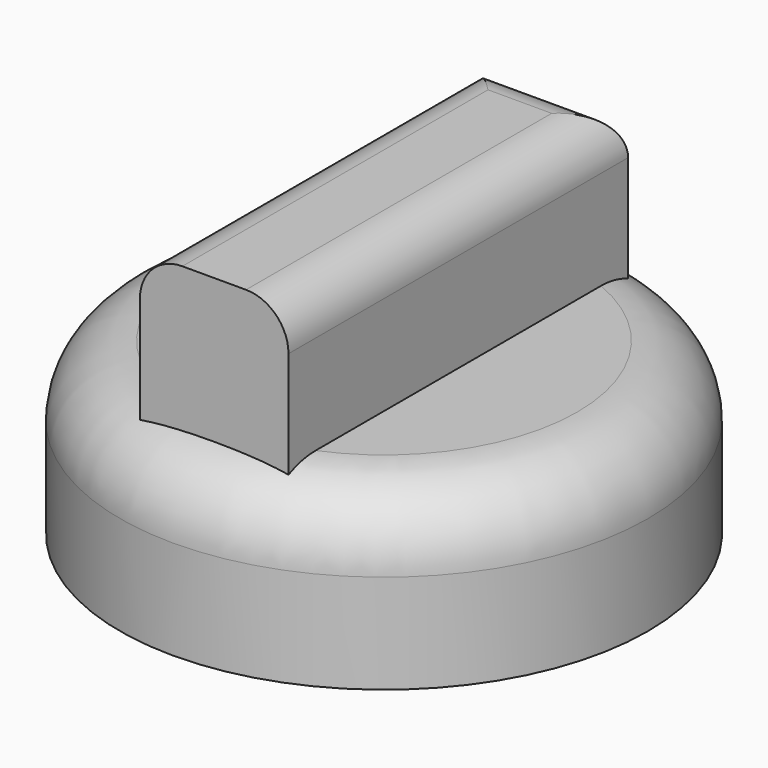
from build123d import *

# Parameters (mm, degrees)
F0_R     = 7
F1_DEPTH = 12
F0_R_2   = 18.6535272591
F2_DEPTH = 12
F3_R     = 5
F5_W     = 10.5
F5_H     = 30
F6_DEPTH = 15
F7_R     = 3


# Not quite as in the source:
# - a feature names something its author has since deleted; it is built from what else it names


with BuildPart() as f1:
    # F0 (on Top) → F1 (new body)
    with BuildSketch(Plane.XY):
        Circle(F0_R)
        Polygon((1.8, 1), (4.5, 1), (4.5, -1), (1.8, -1), (-1.8, -1), (-4.5, -1), (-4.5, 1), (-1.8, 1), (-1.8, 4.32), (1.8, 4.32), align=None, mode=Mode.SUBTRACT)
    extrude(amount=F1_DEPTH)

    # F0 (on Top) → F2 (join)
    with BuildSketch(Plane.XY):
        Circle(F0_R_2)
        Circle(F0_R, mode=Mode.SUBTRACT)
    extrude(amount=F2_DEPTH)

    # F3
    f3_edges = [f1.edges().sort_by_distance(p)[0] for p in [
        (-18.653527, 0, 12),
    ]]
    fillet(f3_edges, radius=F3_R)

    # F5 (on offset) → F6 (join)
    with BuildSketch(Plane.XY.offset(7)):
        Rectangle(F5_W, F5_H)
    extrude(amount=F6_DEPTH)

    # F7
    f7_edges = [f1.edges().sort_by_distance(p)[0] for p in [
        (0, 15, 22),
        (-5.25, 0, 22),
        (5.25, 0, 22),
    ]]
    fillet(f7_edges, radius=F7_R)


solid = f1.part
